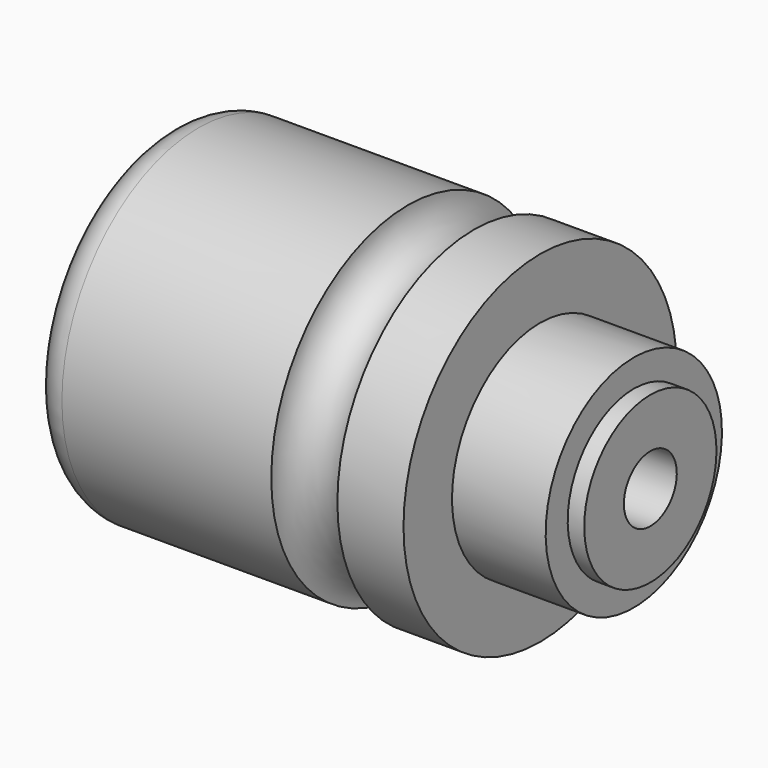
from build123d import *

# Parameters (mm, degrees)
F4_R = 5.99999


# Not quite as in the source:
# - a fillet or chamfer is up to 0.001 mm smaller than in the source, because OpenCascade refuses the exact size


with BuildPart() as f2:
    # F1 (on Front) → F2 (revolve)
    with BuildSketch(Plane.XZ):
        with BuildLine():
            Line((44, 31), (0, 31))
            Line((0, 31), (0, 0))
            Line((0, 0), (88, 0))
            Line((88, 0), (88, 15))
            Line((88, 15), (85, 15))
            Line((85, 15), (85, 20))
            Line((85, 20), (68, 20))
            Line((68, 20), (68, 31))
            Line((68, 31), (56, 31))
            ThreePointArc((56, 31), (50, 25), (44, 31))
        make_face()
    revolve(axis=Axis((48.084679991, 0, 0), (-1, 0, 0)))

    # F0 (on Front) → F3 (revolve, cut)
    with BuildSketch(Plane.XZ):
        Polygon((0, 25), (0, 0), (88, 0), (88, 6), (30, 6), (30, 16), (22, 16), (22, 20.5), (15, 20.5), (15, 12.5), (12, 12.5), (12, 16), (1.5, 16), (1.5, 25), align=None)
    revolve(axis=Axis((-11.2478316676, 0, 0), (-1, 0, 0)), mode=Mode.SUBTRACT)

    # F4 (radius 6 in the source; OpenCascade refuses exactly that, so slightly less here)
    f4_edges = [f2.edges().sort_by_distance(p)[0] for p in [
        (0, 0, -31),
    ]]
    fillet(f4_edges, radius=F4_R)


solid = f2.part
